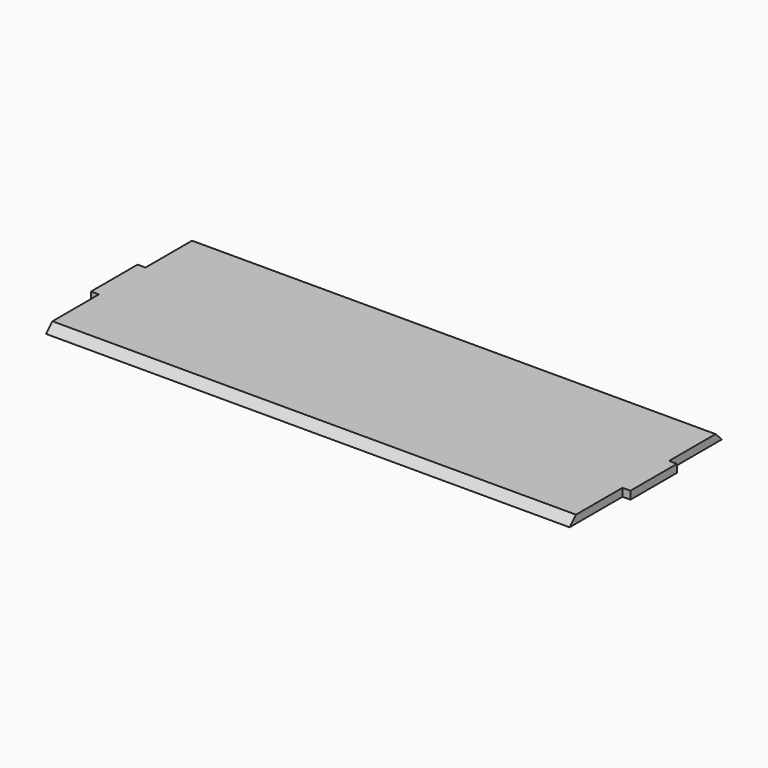
from build123d import *

# Parameters (mm, degrees)
F0_W     = 3
F0_H     = 22
F1_DEPTH = 3
F2_SIZE  = 2.99999


# Not quite as in the source:
# - a fillet or chamfer is up to 0.001 mm smaller than in the source, because OpenCascade refuses the exact size


with BuildPart() as f1:
    # F0 (on Top) → F1 (new body)
    with BuildSketch(Plane.XY):
        Polygon((-79.1548952963, 25), (-79.1548952963, 0), (118.8451047037, 0), (118.8451047037, 25), (118.8451047037, 47), (118.8451047037, 72), (-79.1548952963, 72), (-79.1548952963, 47), align=None)
        with Locations((120.3451047037, 36)):
            Rectangle(F0_W, F0_H)
        with Locations((-80.6548952963, 36)):
            Rectangle(F0_W, F0_H)
    extrude(amount=F1_DEPTH)

    # F2 (size 3 in the source; OpenCascade refuses exactly that, so slightly less here)
    f2_edges = [f1.edges().sort_by_distance(p)[0] for p in [
        (19.845105, 0, 3),
        (19.845105, 72, 3),
    ]]
    chamfer(f2_edges, length=F2_SIZE)


solid = f1.part
